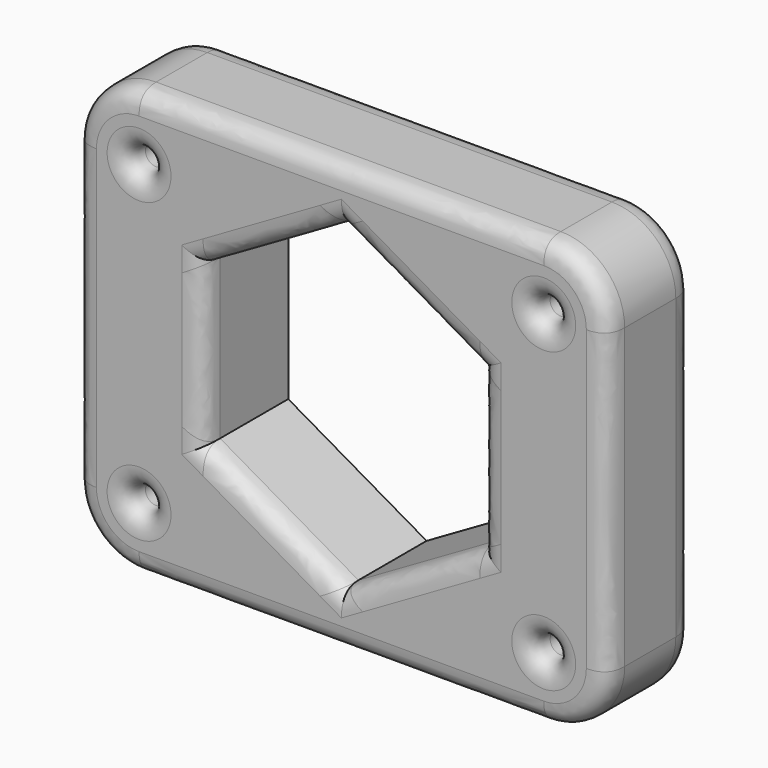
from build123d import *

# Parameters (mm, degrees)
F0_R          = 1
F1_DEPTH      = 10
F2_T1_DEPTH   = 38
F2_T3_DEPTH   = 28
F2_T6_ANGLE   = 90
F2_T8_ANGLE   = 90
F2_T10_ANGLE  = 90
F2_T12_ANGLE  = 90
F2_T20_DEPTH  = 25
F2_T26_DEPTH  = 25
F2_T32_DEPTH  = 25
F2_T38_DEPTH  = 25
F2_T44_DEPTH  = 25
F2_T50_DEPTH  = 25
F2_T58_ANGLE  = 90
F2_T60_ANGLE  = 90
F2_T62_ANGLE  = 90
F2_T64_ANGLE  = 90
F2_T69_DEPTH  = 25
F2_T73_DEPTH  = 25
F2_T80_DEPTH  = 25
F2_T84_DEPTH  = 25
F2_T91_DEPTH  = 25
F2_T95_DEPTH  = 25
F2_T102_DEPTH = 25
F2_T106_DEPTH = 25
F2_T113_DEPTH = 25
F2_T117_DEPTH = 25
F2_T124_DEPTH = 25
F2_T128_DEPTH = 25


# Not quite as in the source:
# - a fillet or chamfer that OpenCascade refuses, or shapes differently, is made with other operations: its cross-section is extruded or revolved along the edge and cut away or added


with BuildPart() as f1:
    # F0 (on Front) → F1 (new body)
    with BuildSketch(Plane.XZ):
        with BuildLine():
            Line((-23.3671131134, -11.5436052999), (14.6328868866, -11.5436052999))
            ThreePointArc((14.6328868866, -11.5436052999), (18.8755275737, -9.7862459871), (20.6328868866, -5.5436052999))
            Line((20.6328868866, -5.5436052999), (20.6328868866, 22.4563947001))
            ThreePointArc((20.6328868866, 22.4563947001), (18.8755275737, 26.6990353872), (14.6328868866, 28.4563947001))
            Line((14.6328868866, 28.4563947001), (-23.3671131134, 28.4563947001))
            ThreePointArc((-23.3671131134, 28.4563947001), (-27.6097538005, 26.6990353872), (-29.3671131134, 22.4563947001))
            Line((-29.3671131134, 22.4563947001), (-29.3671131134, -5.5436052999))
            ThreePointArc((-29.3671131134, -5.5436052999), (-27.6097538005, -9.7862459871), (-23.3671131134, -11.5436052999))
        make_face()
        with Locations((-23.3671131134, -5.5436052999)):
            Circle(F0_R, mode=Mode.SUBTRACT)
        with Locations((14.6328868866, -5.5436052999)):
            Circle(F0_R, mode=Mode.SUBTRACT)
        Polygon((-17.3574941702, 15.9563947001), (-4.3671131134, 23.4563947001), (8.6232679434, 15.9563947001), (8.6232679434, 0.9563947001), (-4.3671131134, -6.5436052999), (-17.3574941702, 0.9563947001), align=None, mode=Mode.SUBTRACT)
        with Locations((-23.3671131134, 22.4563947001)):
            Circle(F0_R, mode=Mode.SUBTRACT)
        with Locations((14.6328868866, 22.4563947001)):
            Circle(F0_R, mode=Mode.SUBTRACT)
    extrude(amount=F1_DEPTH)

    # F2: fillet of radius 2 on 21 edges, made by hand

    # F2_s2 → F2_t1 (cut)
    with BuildSketch(Plane.YZ.offset(-23.3671131134)):
        with BuildLine():
            add(Edge.make_bspline(
                [(-8, -11.5436052999), (-10, -11.5436052999), (-10, -9.5436052999)],
                knots=[0, 0, 0, 1, 1, 1], degree=2, weights=[1, 1, 1]))
            Line((-10, -9.5436052999), (-10, -11.5436052999))
            Line((-10, -11.5436052999), (-8, -11.5436052999))
        make_face()
        with BuildLine():
            add(Edge.make_bspline(
                [(-8, 28.4563947001), (-10, 28.4563947001), (-10, 26.4563947001)],
                knots=[0, 0, 0, 1, 1, 1], degree=2, weights=[1, 1, 1]))
            Line((-10, 26.4563947001), (-10, 28.4563947001))
            Line((-10, 28.4563947001), (-8, 28.4563947001))
        make_face()
        with BuildLine():
            add(Edge.make_bspline(
                [(-2, 28.4563947001), (0, 28.4563947001), (0, 26.4563947001)],
                knots=[0, 0, 0, 1, 1, 1], degree=2, weights=[1, 1, 1]))
            Line((0, 26.4563947001), (0, 28.4563947001))
            Line((0, 28.4563947001), (-2, 28.4563947001))
        make_face()
        with BuildLine():
            add(Edge.make_bspline(
                [(-2, -11.5436052999), (0, -11.5436052999), (0, -9.5436052999)],
                knots=[0, 0, 0, 1, 1, 1], degree=2, weights=[1, 1, 1]))
            Line((0, -9.5436052999), (0, -11.5436052999))
            Line((0, -11.5436052999), (-2, -11.5436052999))
        make_face()
    extrude(amount=F2_T1_DEPTH, mode=Mode.SUBTRACT)

    # F2_s4 → F2_t3 (cut)
    with BuildSketch(Plane.XY.offset(-5.5436052999)):
        with BuildLine():
            add(Edge.make_bspline(
                [(20.6328868866, -8), (20.6328868866, -10), (18.6328868866, -10)],
                knots=[0, 0, 0, 1, 1, 1], degree=2, weights=[1, 1, 1]))
            Line((18.6328868866, -10), (20.6328868866, -10))
            Line((20.6328868866, -10), (20.6328868866, -8))
        make_face()
        with BuildLine():
            add(Edge.make_bspline(
                [(-29.3671131134, -8), (-29.3671131134, -10), (-27.3671131134, -10)],
                knots=[0, 0, 0, 1, 1, 1], degree=2, weights=[1, 1, 1]))
            Line((-27.3671131134, -10), (-29.3671131134, -10))
            Line((-29.3671131134, -10), (-29.3671131134, -8))
        make_face()
        with BuildLine():
            add(Edge.make_bspline(
                [(-29.3671131134, -2), (-29.3671131134, 0), (-27.3671131134, 0)],
                knots=[0, 0, 0, 1, 1, 1], degree=2, weights=[1, 1, 1]))
            Line((-27.3671131134, 0), (-29.3671131134, 0))
            Line((-29.3671131134, 0), (-29.3671131134, -2))
        make_face()
        with BuildLine():
            add(Edge.make_bspline(
                [(20.6328868866, -2), (20.6328868866, 0), (18.6328868866, 0)],
                knots=[0, 0, 0, 1, 1, 1], degree=2, weights=[1, 1, 1]))
            Line((18.6328868866, 0), (20.6328868866, 0))
            Line((20.6328868866, 0), (20.6328868866, -2))
        make_face()
    extrude(amount=F2_T3_DEPTH, mode=Mode.SUBTRACT)

    # F2_s5 → F2_t6 (revolve, cut)
    with BuildSketch(Plane.YZ.offset(14.6328868866)):
        with BuildLine():
            add(Edge.make_bspline(
                [(-8, -11.5436052999), (-10, -11.5436052999), (-10, -9.5436052999)],
                knots=[0, 0, 0, 1, 1, 1], degree=2, weights=[1, 1, 1]))
            Line((-10, -9.5436052999), (-10, -11.5436052999))
            Line((-10, -11.5436052999), (-8, -11.5436052999))
        make_face()
    revolve(axis=Axis((14.6328868866, -10, -5.5436052999), (0, -1, 0)), revolution_arc=F2_T6_ANGLE, mode=Mode.SUBTRACT)

    # F2_s7 → F2_t8 (revolve, cut)
    with BuildSketch(Plane.XY.offset(22.4563947001)):
        with BuildLine():
            add(Edge.make_bspline(
                [(20.6328868866, -8), (20.6328868866, -10), (18.6328868866, -10)],
                knots=[0, 0, 0, 1, 1, 1], degree=2, weights=[1, 1, 1]))
            Line((18.6328868866, -10), (20.6328868866, -10))
            Line((20.6328868866, -10), (20.6328868866, -8))
        make_face()
    revolve(axis=Axis((14.6328868866, -10, 22.4563947001), (0, -1, 0)), revolution_arc=F2_T8_ANGLE, mode=Mode.SUBTRACT)

    # F2_s9 → F2_t10 (revolve, cut)
    with BuildSketch(Plane.YZ.offset(-23.3671131134)):
        with BuildLine():
            add(Edge.make_bspline(
                [(-8, 28.4563947001), (-10, 28.4563947001), (-10, 26.4563947001)],
                knots=[0, 0, 0, 1, 1, 1], degree=2, weights=[1, 1, 1]))
            Line((-10, 26.4563947001), (-10, 28.4563947001))
            Line((-10, 28.4563947001), (-8, 28.4563947001))
        make_face()
    revolve(axis=Axis((-23.3671131134, -10, 22.4563947001), (0, -1, 0)), revolution_arc=F2_T10_ANGLE, mode=Mode.SUBTRACT)

    # F2_s11 → F2_t12 (revolve, cut)
    with BuildSketch(Plane.XY.offset(-5.5436052999)):
        with BuildLine():
            add(Edge.make_bspline(
                [(-29.3671131134, -8), (-29.3671131134, -10), (-27.3671131134, -10)],
                knots=[0, 0, 0, 1, 1, 1], degree=2, weights=[1, 1, 1]))
            Line((-27.3671131134, -10), (-29.3671131134, -10))
            Line((-29.3671131134, -10), (-29.3671131134, -8))
        make_face()
    revolve(axis=Axis((-23.3671131134, -10, -5.5436052999), (0, -1, 0)), revolution_arc=F2_T12_ANGLE, mode=Mode.SUBTRACT)

    # F2_s13 → F2_t14 (revolve, cut)
    with BuildSketch(Plane.XY.offset(-5.5436052999)):
        with BuildLine():
            add(Edge.make_bspline(
                [(-22.3671131134, -8), (-22.3671131134, -10), (-20.3671131134, -10)],
                knots=[0, 0, 0, 1, 1, 1], degree=2, weights=[1, 1, 1]))
            Line((-20.3671131134, -10), (-22.3671131134, -10))
            Line((-22.3671131134, -10), (-22.3671131134, -8))
        make_face()
    revolve(axis=Axis((-23.3671131134, -10, -5.5436052999), (0, -1, 0)), mode=Mode.SUBTRACT)

    # F2_s15 → F2_t16 (revolve, cut)
    with BuildSketch(Plane.XY.offset(-5.5436052999)):
        with BuildLine():
            add(Edge.make_bspline(
                [(15.6328868866, -8), (15.6328868866, -10), (17.6328868866, -10)],
                knots=[0, 0, 0, 1, 1, 1], degree=2, weights=[1, 1, 1]))
            Line((17.6328868866, -10), (15.6328868866, -10))
            Line((15.6328868866, -10), (15.6328868866, -8))
        make_face()
    revolve(axis=Axis((14.6328868866, -10, -5.5436052999), (0, -1, 0)), mode=Mode.SUBTRACT)


with BuildPart() as f2_tool18:
    # F2_s19 → F2_t20 (new body)
    with BuildSketch(Plane(origin=(3.8882563949, 0, -2.2448858763), x_dir=(0, 1, 0), z_dir=(-0.8660254038, 0, 0.5))):
        with BuildLine():
            add(Edge.make_bspline(
                [(-8, 7.8504849788), (-10, 7.8504849788), (-10, 9.8504849788)],
                knots=[0, 0, 0, 1, 1, 1], degree=2, weights=[1, 1, 1]))
            Line((-10, 9.8504849788), (-10, 7.8504849788))
            Line((-10, 7.8504849788), (-8, 7.8504849788))
        make_face()
    extrude(amount=F2_T20_DEPTH)

    split(bisect_by=Plane(origin=(1.7416859327, 0, -3.0166885263), x_dir=(0, 1, 0), z_dir=(-0.5, 0, 0.8660254038)), keep=Keep.TOP)

    split(bisect_by=Plane.YZ.offset(-17.3574941702), keep=Keep.TOP)


with BuildPart() as f1_1:
    add(f1.part)

    # F2_t17: cut F2_tool18
    add(f2_tool18.part, mode=Mode.SUBTRACT)


with BuildPart() as f2_tool24:
    # F2_s25 → F2_t26 (new body)
    with BuildSketch(Plane.XY.offset(-4.0436052999)):
        with BuildLine():
            add(Edge.make_bspline(
                [(-17.3574941702, -8), (-17.3574941702, -10), (-19.3574941702, -10)],
                knots=[0, 0, 0, 1, 1, 1], degree=2, weights=[1, 1, 1]))
            Line((-19.3574941702, -10), (-17.3574941702, -10))
            Line((-17.3574941702, -10), (-17.3574941702, -8))
        make_face()
    extrude(amount=F2_T26_DEPTH)

    split(bisect_by=Plane(origin=(-3.9252424894, 0, -6.7987194237), x_dir=(0, 1, 0), z_dir=(0.5, 0, 0.8660254038)), keep=Keep.TOP)

    split(bisect_by=Plane(origin=(-11.2486951241, 0, 19.4833114737), x_dir=(0, 1, 0), z_dir=(0.5, 0, -0.8660254038)), keep=Keep.TOP)


with BuildPart() as f1_2:
    add(f1_1.part)

    # F2_t23: cut F2_tool24
    add(f2_tool24.part, mode=Mode.SUBTRACT)


with BuildPart() as f2_tool30:
    # F2_s31 → F2_t32 (new body)
    with BuildSketch(Plane(origin=(-10.438926065, 0, -6.0269167737), x_dir=(0, 1, 0), z_dir=(0.8660254038, 0, 0.5))):
        with BuildLine():
            add(Edge.make_bspline(
                [(-8, 22.4973902481), (-10, 22.4973902481), (-10, 24.4973902481)],
                knots=[0, 0, 0, 1, 1, 1], degree=2, weights=[1, 1, 1]))
            Line((-10, 24.4973902481), (-10, 22.4973902481))
            Line((-10, 22.4973902481), (-8, 22.4973902481))
        make_face()
    extrude(amount=F2_T32_DEPTH)

    split(bisect_by=Plane.YZ.offset(-17.3574941702), keep=Keep.TOP)

    split(bisect_by=Plane(origin=(9.0651385674, 0, 15.7012805763), x_dir=(0, 1, 0), z_dir=(-0.5, 0, -0.8660254038)), keep=Keep.TOP)


with BuildPart() as f1_3:
    add(f1_2.part)

    # F2_t29: cut F2_tool30
    add(f2_tool30.part, mode=Mode.SUBTRACT)


with BuildPart() as f2_tool36:
    # F2_s37 → F2_t38 (new body)
    with BuildSketch(Plane(origin=(-17.7623786997, 0, 10.2551141237), x_dir=(0, 1, 0), z_dir=(0.8660254038, 0, -0.5))):
        with BuildLine():
            add(Edge.make_bspline(
                [(-8, 18.1302771347), (-10, 18.1302771347), (-10, 20.1302771347)],
                knots=[0, 0, 0, 1, 1, 1], degree=2, weights=[1, 1, 1]))
            Line((-10, 20.1302771347), (-10, 18.1302771347))
            Line((-10, 18.1302771347), (-8, 18.1302771347))
        make_face()
    extrude(amount=F2_T38_DEPTH)

    split(bisect_by=Plane(origin=(-11.2486951241, 0, 19.4833114737), x_dir=(0, 1, 0), z_dir=(0.5, 0, -0.8660254038)), keep=Keep.TOP)

    split(bisect_by=Plane.YZ.offset(8.6232679434), keep=Keep.BOTTOM)


with BuildPart() as f1_4:
    add(f1_3.part)

    # F2_t35: cut F2_tool36
    add(f2_tool36.part, mode=Mode.SUBTRACT)


with BuildPart() as f2_tool42:
    # F2_s43 → F2_t44 (new body)
    with BuildSketch(Plane.XY.offset(20.9563947001)):
        with BuildLine():
            add(Edge.make_bspline(
                [(8.6232679434, -8), (8.6232679434, -10), (10.6232679434, -10)],
                knots=[0, 0, 0, 1, 1, 1], degree=2, weights=[1, 1, 1]))
            Line((10.6232679434, -10), (8.6232679434, -10))
            Line((8.6232679434, -10), (8.6232679434, -8))
        make_face()
    extrude(amount=-F2_T44_DEPTH)

    split(bisect_by=Plane(origin=(9.0651385674, 0, 15.7012805763), x_dir=(0, 1, 0), z_dir=(-0.5, 0, -0.8660254038)), keep=Keep.TOP)

    split(bisect_by=Plane(origin=(1.7416859327, 0, -3.0166885263), x_dir=(0, 1, 0), z_dir=(-0.5, 0, 0.8660254038)), keep=Keep.TOP)


with BuildPart() as f1_5:
    add(f1_4.part)

    # F2_t41: cut F2_tool42
    add(f2_tool42.part, mode=Mode.SUBTRACT)


with BuildPart() as f2_tool48:
    # F2_s49 → F2_t50 (new body)
    with BuildSketch(Plane(origin=(11.2117090296, 0, 6.4730832263), x_dir=(0, 1, 0), z_dir=(-0.8660254038, 0, -0.5))):
        with BuildLine():
            add(Edge.make_bspline(
                [(-8, 3.4833718654), (-10, 3.4833718654), (-10, 5.4833718654)],
                knots=[0, 0, 0, 1, 1, 1], degree=2, weights=[1, 1, 1]))
            Line((-10, 5.4833718654), (-10, 3.4833718654))
            Line((-10, 3.4833718654), (-8, 3.4833718654))
        make_face()
    extrude(amount=F2_T50_DEPTH)

    split(bisect_by=Plane(origin=(-3.9252424894, 0, -6.7987194237), x_dir=(0, 1, 0), z_dir=(0.5, 0, 0.8660254038)), keep=Keep.TOP)

    split(bisect_by=Plane.YZ.offset(8.6232679434), keep=Keep.BOTTOM)


with BuildPart() as f1_6:
    add(f1_5.part)

    # F2_t47: cut F2_tool48
    add(f2_tool48.part, mode=Mode.SUBTRACT)

    # F2_s53 → F2_t54 (revolve, cut)
    with BuildSketch(Plane.XY.offset(22.4563947001)):
        with BuildLine():
            add(Edge.make_bspline(
                [(-22.3671131134, -8), (-22.3671131134, -10), (-20.3671131134, -10)],
                knots=[0, 0, 0, 1, 1, 1], degree=2, weights=[1, 1, 1]))
            Line((-20.3671131134, -10), (-22.3671131134, -10))
            Line((-22.3671131134, -10), (-22.3671131134, -8))
        make_face()
    revolve(axis=Axis((-23.3671131134, -10, 22.4563947001), (0, -1, 0)), mode=Mode.SUBTRACT)

    # F2_s55 → F2_t56 (revolve, cut)
    with BuildSketch(Plane.XY.offset(22.4563947001)):
        with BuildLine():
            add(Edge.make_bspline(
                [(15.6328868866, -8), (15.6328868866, -10), (17.6328868866, -10)],
                knots=[0, 0, 0, 1, 1, 1], degree=2, weights=[1, 1, 1]))
            Line((17.6328868866, -10), (15.6328868866, -10))
            Line((15.6328868866, -10), (15.6328868866, -8))
        make_face()
    revolve(axis=Axis((14.6328868866, -10, 22.4563947001), (0, -1, 0)), mode=Mode.SUBTRACT)

    # F2_s57 → F2_t58 (revolve, cut)
    with BuildSketch(Plane.XY.offset(22.4563947001)):
        with BuildLine():
            add(Edge.make_bspline(
                [(20.6328868866, -2), (20.6328868866, 0), (18.6328868866, 0)],
                knots=[0, 0, 0, 1, 1, 1], degree=2, weights=[1, 1, 1]))
            Line((18.6328868866, 0), (20.6328868866, 0))
            Line((20.6328868866, 0), (20.6328868866, -2))
        make_face()
    revolve(axis=Axis((14.6328868866, 0, 22.4563947001), (0, -1, 0)), revolution_arc=F2_T58_ANGLE, mode=Mode.SUBTRACT)

    # F2_s59 → F2_t60 (revolve, cut)
    with BuildSketch(Plane.YZ.offset(-23.3671131134)):
        with BuildLine():
            add(Edge.make_bspline(
                [(-2, 28.4563947001), (0, 28.4563947001), (0, 26.4563947001)],
                knots=[0, 0, 0, 1, 1, 1], degree=2, weights=[1, 1, 1]))
            Line((0, 26.4563947001), (0, 28.4563947001))
            Line((0, 28.4563947001), (-2, 28.4563947001))
        make_face()
    revolve(axis=Axis((-23.3671131134, 0, 22.4563947001), (0, -1, 0)), revolution_arc=F2_T60_ANGLE, mode=Mode.SUBTRACT)

    # F2_s61 → F2_t62 (revolve, cut)
    with BuildSketch(Plane.XY.offset(-5.5436052999)):
        with BuildLine():
            add(Edge.make_bspline(
                [(-29.3671131134, -2), (-29.3671131134, 0), (-27.3671131134, 0)],
                knots=[0, 0, 0, 1, 1, 1], degree=2, weights=[1, 1, 1]))
            Line((-27.3671131134, 0), (-29.3671131134, 0))
            Line((-29.3671131134, 0), (-29.3671131134, -2))
        make_face()
    revolve(axis=Axis((-23.3671131134, 0, -5.5436052999), (0, -1, 0)), revolution_arc=F2_T62_ANGLE, mode=Mode.SUBTRACT)

    # F2_s63 → F2_t64 (revolve, cut)
    with BuildSketch(Plane.YZ.offset(14.6328868866)):
        with BuildLine():
            add(Edge.make_bspline(
                [(-2, -11.5436052999), (0, -11.5436052999), (0, -9.5436052999)],
                knots=[0, 0, 0, 1, 1, 1], degree=2, weights=[1, 1, 1]))
            Line((0, -9.5436052999), (0, -11.5436052999))
            Line((0, -11.5436052999), (-2, -11.5436052999))
        make_face()
    revolve(axis=Axis((14.6328868866, 0, -5.5436052999), (0, -1, 0)), revolution_arc=F2_T64_ANGLE, mode=Mode.SUBTRACT)


with BuildPart() as f2_tool67:
    # F2_s68 → F2_t69 (new body)
    with BuildSketch(Plane(origin=(3.8882563949, 0, -2.2448858763), x_dir=(0, 1, 0), z_dir=(-0.8660254038, 0, 0.5))):
        with BuildLine():
            add(Edge.make_bspline(
                [(-8, 7.8504849788), (-10, 7.8504849788), (-10, 9.8504849788)],
                knots=[0, 0, 0, 1, 1, 1], degree=2, weights=[1, 1, 1]))
            Line((-10, 9.8504849788), (-10, 7.8504849788))
            Line((-10, 7.8504849788), (-8, 7.8504849788))
        make_face()
    extrude(amount=F2_T69_DEPTH)

    split(bisect_by=Plane(origin=(1.7416859327, 0, -3.0166885263), x_dir=(0, 1, 0), z_dir=(0.5, 0, -0.8660254038)), keep=Keep.TOP)


with BuildPart() as f2_tool71:
    # F2_s72 → F2_t73 (new body)
    with BuildSketch(Plane(origin=(11.2117090296, 0, 6.4730832263), x_dir=(0, 1, 0), z_dir=(-0.8660254038, 0, -0.5))):
        with BuildLine():
            add(Edge.make_bspline(
                [(-8, 3.4833718654), (-10, 3.4833718654), (-10, 5.4833718654)],
                knots=[0, 0, 0, 1, 1, 1], degree=2, weights=[1, 1, 1]))
            Line((-10, 5.4833718654), (-10, 3.4833718654))
            Line((-10, 3.4833718654), (-8, 3.4833718654))
        make_face()
    extrude(amount=F2_T73_DEPTH)

    split(bisect_by=Plane(origin=(-3.9252424894, 0, -6.7987194237), x_dir=(0, 1, 0), z_dir=(-0.5, 0, -0.8660254038)), keep=Keep.TOP)


with BuildPart() as f2_tool67_1:
    add(f2_tool67.part)

    # F2_t75: intersect F2_tool71
    add(f2_tool71.part, mode=Mode.INTERSECT)


with BuildPart() as f1_7:
    add(f1_6.part)

    # F2_t65: cut F2_tool67
    add(f2_tool67_1.part, mode=Mode.SUBTRACT)


with BuildPart() as f2_tool78:
    # F2_s79 → F2_t80 (new body)
    with BuildSketch(Plane(origin=(3.8882563949, 0, -2.2448858763), x_dir=(0, 1, 0), z_dir=(-0.8660254038, 0, 0.5))):
        with BuildLine():
            add(Edge.make_bspline(
                [(-8, 7.8504849788), (-10, 7.8504849788), (-10, 9.8504849788)],
                knots=[0, 0, 0, 1, 1, 1], degree=2, weights=[1, 1, 1]))
            Line((-10, 9.8504849788), (-10, 7.8504849788))
            Line((-10, 7.8504849788), (-8, 7.8504849788))
        make_face()
    extrude(amount=F2_T80_DEPTH)

    split(bisect_by=Plane.YZ.offset(-17.3574941702), keep=Keep.BOTTOM)


with BuildPart() as f2_tool82:
    # F2_s83 → F2_t84 (new body)
    with BuildSketch(Plane.XY.offset(-4.0436052999)):
        with BuildLine():
            add(Edge.make_bspline(
                [(-17.3574941702, -8), (-17.3574941702, -10), (-19.3574941702, -10)],
                knots=[0, 0, 0, 1, 1, 1], degree=2, weights=[1, 1, 1]))
            Line((-19.3574941702, -10), (-17.3574941702, -10))
            Line((-17.3574941702, -10), (-17.3574941702, -8))
        make_face()
    extrude(amount=F2_T84_DEPTH)

    split(bisect_by=Plane(origin=(-3.9252424894, 0, -6.7987194237), x_dir=(0, 1, 0), z_dir=(-0.5, 0, -0.8660254038)), keep=Keep.TOP)


with BuildPart() as f2_tool78_1:
    add(f2_tool78.part)

    # F2_t86: intersect F2_tool82
    add(f2_tool82.part, mode=Mode.INTERSECT)


with BuildPart() as f1_8:
    add(f1_7.part)

    # F2_t76: cut F2_tool78
    add(f2_tool78_1.part, mode=Mode.SUBTRACT)


with BuildPart() as f2_tool89:
    # F2_s90 → F2_t91 (new body)
    with BuildSketch(Plane.XY.offset(-4.0436052999)):
        with BuildLine():
            add(Edge.make_bspline(
                [(-17.3574941702, -8), (-17.3574941702, -10), (-19.3574941702, -10)],
                knots=[0, 0, 0, 1, 1, 1], degree=2, weights=[1, 1, 1]))
            Line((-19.3574941702, -10), (-17.3574941702, -10))
            Line((-17.3574941702, -10), (-17.3574941702, -8))
        make_face()
    extrude(amount=F2_T91_DEPTH)

    split(bisect_by=Plane(origin=(-11.2486951241, 0, 19.4833114737), x_dir=(0, 1, 0), z_dir=(-0.5, 0, 0.8660254038)), keep=Keep.TOP)


with BuildPart() as f2_tool93:
    # F2_s94 → F2_t95 (new body)
    with BuildSketch(Plane(origin=(-10.438926065, 0, -6.0269167737), x_dir=(0, 1, 0), z_dir=(0.8660254038, 0, 0.5))):
        with BuildLine():
            add(Edge.make_bspline(
                [(-8, 22.4973902481), (-10, 22.4973902481), (-10, 24.4973902481)],
                knots=[0, 0, 0, 1, 1, 1], degree=2, weights=[1, 1, 1]))
            Line((-10, 24.4973902481), (-10, 22.4973902481))
            Line((-10, 22.4973902481), (-8, 22.4973902481))
        make_face()
    extrude(amount=F2_T95_DEPTH)

    split(bisect_by=Plane.YZ.offset(-17.3574941702), keep=Keep.BOTTOM)


with BuildPart() as f2_tool89_1:
    add(f2_tool89.part)

    # F2_t97: intersect F2_tool93
    add(f2_tool93.part, mode=Mode.INTERSECT)


with BuildPart() as f1_9:
    add(f1_8.part)

    # F2_t87: cut F2_tool89
    add(f2_tool89_1.part, mode=Mode.SUBTRACT)


with BuildPart() as f2_tool100:
    # F2_s101 → F2_t102 (new body)
    with BuildSketch(Plane(origin=(-10.438926065, 0, -6.0269167737), x_dir=(0, 1, 0), z_dir=(0.8660254038, 0, 0.5))):
        with BuildLine():
            add(Edge.make_bspline(
                [(-8, 22.4973902481), (-10, 22.4973902481), (-10, 24.4973902481)],
                knots=[0, 0, 0, 1, 1, 1], degree=2, weights=[1, 1, 1]))
            Line((-10, 24.4973902481), (-10, 22.4973902481))
            Line((-10, 22.4973902481), (-8, 22.4973902481))
        make_face()
    extrude(amount=F2_T102_DEPTH)

    split(bisect_by=Plane(origin=(9.0651385674, 0, 15.7012805763), x_dir=(0, 1, 0), z_dir=(0.5, 0, 0.8660254038)), keep=Keep.TOP)


with BuildPart() as f2_tool104:
    # F2_s105 → F2_t106 (new body)
    with BuildSketch(Plane(origin=(-17.7623786997, 0, 10.2551141237), x_dir=(0, 1, 0), z_dir=(0.8660254038, 0, -0.5))):
        with BuildLine():
            add(Edge.make_bspline(
                [(-8, 18.1302771347), (-10, 18.1302771347), (-10, 20.1302771347)],
                knots=[0, 0, 0, 1, 1, 1], degree=2, weights=[1, 1, 1]))
            Line((-10, 20.1302771347), (-10, 18.1302771347))
            Line((-10, 18.1302771347), (-8, 18.1302771347))
        make_face()
    extrude(amount=F2_T106_DEPTH)

    split(bisect_by=Plane(origin=(-11.2486951241, 0, 19.4833114737), x_dir=(0, 1, 0), z_dir=(-0.5, 0, 0.8660254038)), keep=Keep.TOP)


with BuildPart() as f2_tool100_1:
    add(f2_tool100.part)

    # F2_t108: intersect F2_tool104
    add(f2_tool104.part, mode=Mode.INTERSECT)


with BuildPart() as f1_10:
    add(f1_9.part)

    # F2_t98: cut F2_tool100
    add(f2_tool100_1.part, mode=Mode.SUBTRACT)


with BuildPart() as f2_tool111:
    # F2_s112 → F2_t113 (new body)
    with BuildSketch(Plane(origin=(-17.7623786997, 0, 10.2551141237), x_dir=(0, 1, 0), z_dir=(0.8660254038, 0, -0.5))):
        with BuildLine():
            add(Edge.make_bspline(
                [(-8, 18.1302771347), (-10, 18.1302771347), (-10, 20.1302771347)],
                knots=[0, 0, 0, 1, 1, 1], degree=2, weights=[1, 1, 1]))
            Line((-10, 20.1302771347), (-10, 18.1302771347))
            Line((-10, 18.1302771347), (-8, 18.1302771347))
        make_face()
    extrude(amount=F2_T113_DEPTH)

    split(bisect_by=Plane.YZ.offset(8.6232679434), keep=Keep.TOP)


with BuildPart() as f2_tool115:
    # F2_s116 → F2_t117 (new body)
    with BuildSketch(Plane.XY.offset(20.9563947001)):
        with BuildLine():
            add(Edge.make_bspline(
                [(8.6232679434, -8), (8.6232679434, -10), (10.6232679434, -10)],
                knots=[0, 0, 0, 1, 1, 1], degree=2, weights=[1, 1, 1]))
            Line((10.6232679434, -10), (8.6232679434, -10))
            Line((8.6232679434, -10), (8.6232679434, -8))
        make_face()
    extrude(amount=-F2_T117_DEPTH)

    split(bisect_by=Plane(origin=(9.0651385674, 0, 15.7012805763), x_dir=(0, 1, 0), z_dir=(0.5, 0, 0.8660254038)), keep=Keep.TOP)


with BuildPart() as f2_tool111_1:
    add(f2_tool111.part)

    # F2_t119: intersect F2_tool115
    add(f2_tool115.part, mode=Mode.INTERSECT)


with BuildPart() as f1_11:
    add(f1_10.part)

    # F2_t109: cut F2_tool111
    add(f2_tool111_1.part, mode=Mode.SUBTRACT)


with BuildPart() as f2_tool122:
    # F2_s123 → F2_t124 (new body)
    with BuildSketch(Plane.XY.offset(20.9563947001)):
        with BuildLine():
            add(Edge.make_bspline(
                [(8.6232679434, -8), (8.6232679434, -10), (10.6232679434, -10)],
                knots=[0, 0, 0, 1, 1, 1], degree=2, weights=[1, 1, 1]))
            Line((10.6232679434, -10), (8.6232679434, -10))
            Line((8.6232679434, -10), (8.6232679434, -8))
        make_face()
    extrude(amount=-F2_T124_DEPTH)

    split(bisect_by=Plane(origin=(1.7416859327, 0, -3.0166885263), x_dir=(0, 1, 0), z_dir=(0.5, 0, -0.8660254038)), keep=Keep.TOP)


with BuildPart() as f2_tool126:
    # F2_s127 → F2_t128 (new body)
    with BuildSketch(Plane(origin=(11.2117090296, 0, 6.4730832263), x_dir=(0, 1, 0), z_dir=(-0.8660254038, 0, -0.5))):
        with BuildLine():
            add(Edge.make_bspline(
                [(-8, 3.4833718654), (-10, 3.4833718654), (-10, 5.4833718654)],
                knots=[0, 0, 0, 1, 1, 1], degree=2, weights=[1, 1, 1]))
            Line((-10, 5.4833718654), (-10, 3.4833718654))
            Line((-10, 3.4833718654), (-8, 3.4833718654))
        make_face()
    extrude(amount=F2_T128_DEPTH)

    split(bisect_by=Plane.YZ.offset(8.6232679434), keep=Keep.TOP)


with BuildPart() as f2_tool122_1:
    add(f2_tool122.part)

    # F2_t130: intersect F2_tool126
    add(f2_tool126.part, mode=Mode.INTERSECT)


with BuildPart() as f1_12:
    add(f1_11.part)

    # F2_t120: cut F2_tool122
    add(f2_tool122_1.part, mode=Mode.SUBTRACT)


solid = f1_12.part
